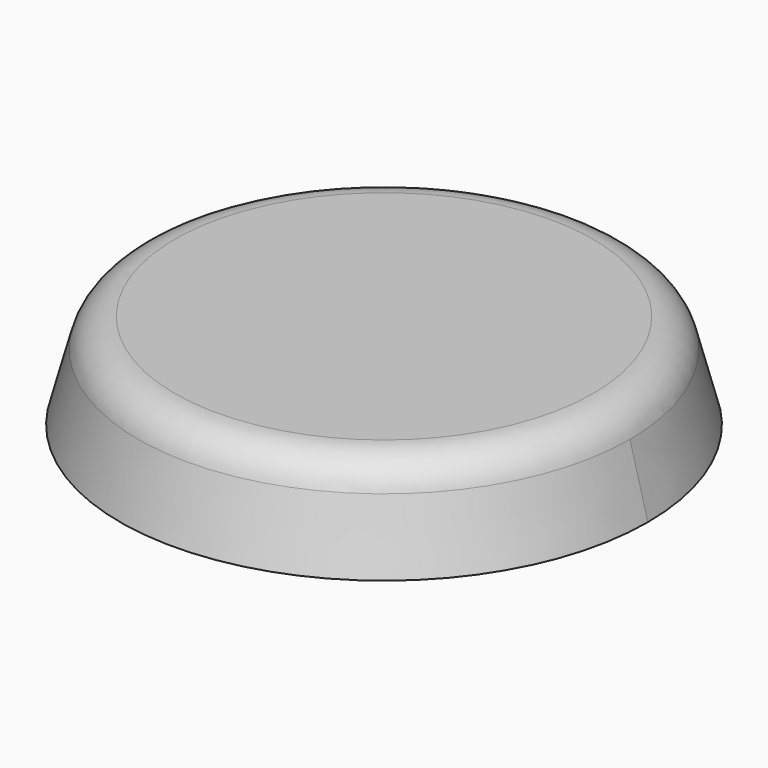
from build123d import *
from build123d import SkipClean  # not in build123d's __all__

# Parameters (mm, degrees)
F0_R     = 12.5
F1_DEPTH = 5
F1_TAPER = -15
F2_R     = 2
F4_DEPTH = 25
F5_R     = 1


with BuildPart() as f1:
    # F0 (on Top) → F1 (new body)
    with BuildSketch(Plane.XY):
        Circle(F0_R)
    extrude(amount=-F1_DEPTH, taper=F1_TAPER)

    # F2
    f2_edges = [f1.edges().sort_by_distance(p)[0] for p in [
        (-12.5, 0, 0),
    ]]
    fillet(f2_edges, radius=F2_R)

    # F3 (on Top) → F4 (cut)
    with BuildSketch(Plane.XY):
        with BuildLine():
            ThreePointArc((1.5, 13.7582182094), (0, 13.8397459622), (-1.5, 13.7582182094))
            Line((-1.5, 13.7582182094), (-1, 12.8971976766))
            Line((-1, 12.8971976766), (1, 12.8971976766))
            Line((1, 12.8971976766), (1.5, 13.7582182094))
        make_face()
    with SkipClean():  # cleaning this boolean's faces spoils the solid; the shape is the same uncleaned
        extrude(amount=-F4_DEPTH, mode=Mode.SUBTRACT)

    # F5
    f5_edges = [f1.edges().sort_by_distance(p)[0] for p in [
        (-1, 12.897198, -3.313415),
        (1, 12.897198, -3.313415),
    ]]
    fillet(f5_edges, radius=F5_R)


solid = f1.part
